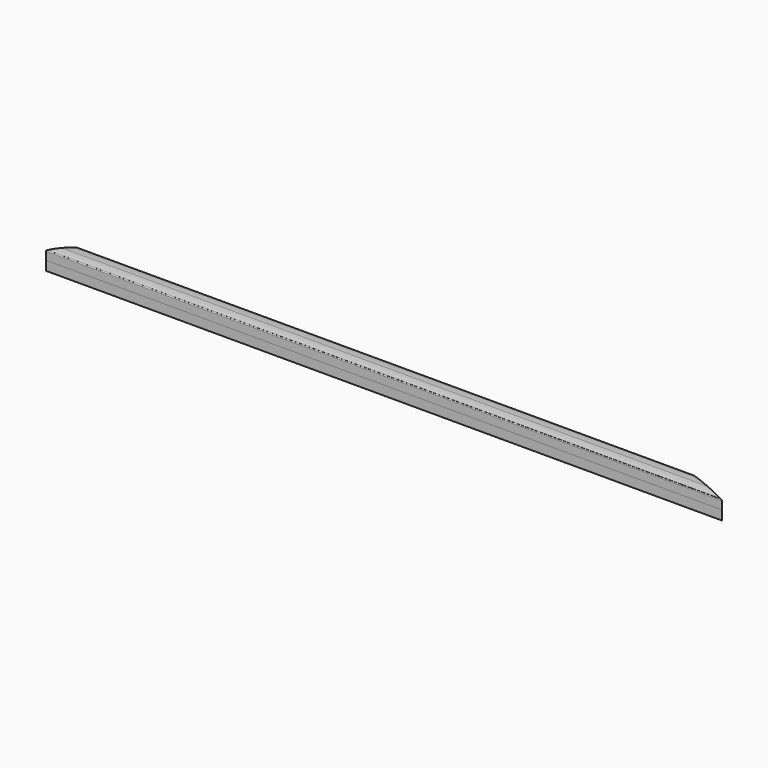
from build123d import *

# Parameters (mm, degrees)
F2_DEPTH      = 1000
F4_DEPTH      = 1000
F8_DEPTH      = 10.001
F8_DEPTH_BACK = 10.001


# Not quite as in the source:
# - ends of sketch curves that miss each other by under 0.0002 mm in the source are joined


with BuildPart() as f2:
    # F1 (on Right) → F2 (new body)
    with BuildSketch(Plane.YZ):
        with BuildLine():
            Line((0, -9), (0, -10))
            Line((0, -10), (10, -10))
            Line((10, -10), (10, -0.2))
            Line((10, -0.2), (9, -0.2))
            ThreePointArc((9, -0.2), (8.5, -0.7), (9, -1.2))
            ThreePointArc((9, -1.2), (9.5, -1.7), (9, -2.2))
            Line((9, -2.2), (9, -9))
            Line((9, -9), (0, -9))
        make_face()
    extrude(amount=F2_DEPTH)

    # F5: F2 across plane


with BuildPart() as f4:
    # F3 (on Right) → F4 (new body)
    with BuildSketch(Plane.YZ):
        with BuildLine():
            Line((9, -0.2), (10, -0.2))
            Line((10, -0.2), (10, 8.1663783152))
            ThreePointArc((10, 8.1663783152), (9.7693092582, 8.8052548802), (9.1836734694, 9.1493656277))
            ThreePointArc((9.1836734694, 9.1493656277), (4.6114920912, 9.7868872364), (0, 10))
            Line((0, 10), (0, 9))
            ThreePointArc((0, 9), (4.5192622493, 8.7911494917), (9, 8.1663783152))
            Line((9, 8.1663783152), (9, 0.8))
            ThreePointArc((9, 0.8), (7.5, -0.7), (9, -2.2))
            ThreePointArc((9, -2.2), (9.5, -1.7), (9, -1.2))
            ThreePointArc((9, -1.2), (8.5, -0.7), (9, -0.2))
        make_face()
    extrude(amount=F4_DEPTH)

    # F6: F4 across plane


with BuildPart() as f2_1:
    add(f2.part)
    add(f2.part.mirror(Plane.XZ))


with BuildPart() as f4_1:
    add(f4.part)
    add(f4.part.mirror(Plane.XZ))


with BuildPart() as f8_tool:
    # F7 (on Top) → F8 (new body, two sides)
    with BuildSketch(Plane.XY) as f8_sk:
        Polygon((0, 10), (0, 0), (0, -10), (17.3857347563, 10), align=None)
        Polygon((664.0031490553, 10), (710, -10), (1016.9613361359, -10), (1016.9613361359, 10), (709.9114895723, 10), align=None)
    extrude(amount=F8_DEPTH)
    extrude(f8_sk.sketch, amount=-F8_DEPTH_BACK)


with BuildPart() as f2_2:
    add(f2_1.part)

    # F8: cut by f8_tool
    add(f8_tool.part, mode=Mode.SUBTRACT)


with BuildPart() as f4_2:
    add(f4_1.part)

    # F8: cut by f8_tool
    add(f8_tool.part, mode=Mode.SUBTRACT)


solid = Compound([f2_2.part, f4_2.part])
